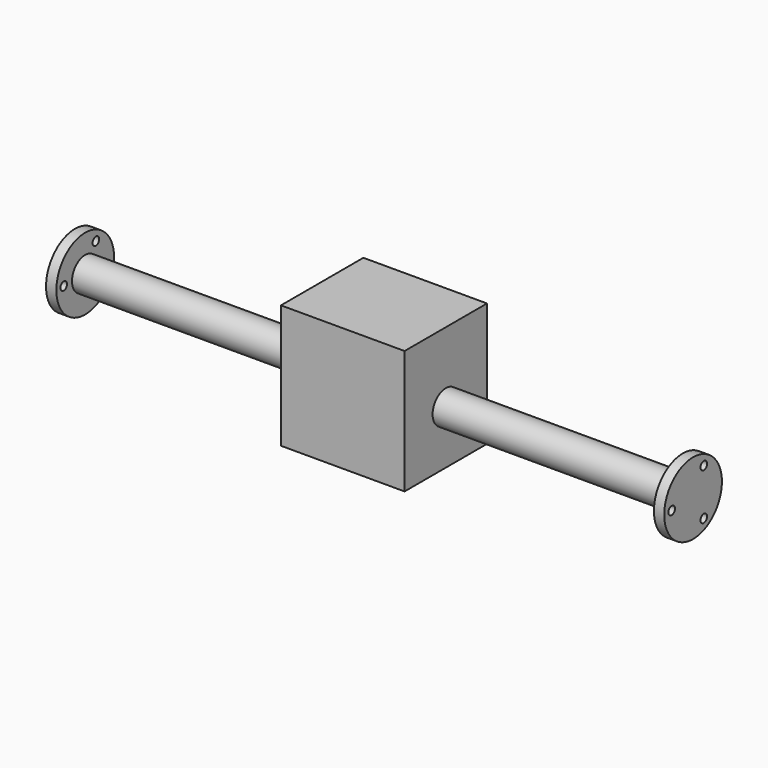
from build123d import *

# Parameters (mm, degrees)
F1_R            = 17.5
F2_DEPTH        = 5
F3_W            = 50
F3_H            = 60
F4_DEPTH        = 30
F5_R            = 8
F6_DEPTH        = 115
F7_R            = 2
F8_DEPTH        = 25
F8_COPIES_COUNT = 3


# Not quite as in the source:
# - a pattern or mirror of a feature is missing from the dataset's text; its kind, count and spacing are read off the source's solid


with BuildPart() as f2:
    # F1 (on offset) → F2 (new body)
    with BuildSketch(Plane.YZ.offset(150)):
        Circle(F1_R)
    extrude(amount=-F2_DEPTH)



with BuildPart() as f4:
    # F3 (on Right) → F4 (new body)
    with BuildSketch(Plane.YZ):
        with Locations((0, 4)):
            Rectangle(F3_W, F3_H)
    extrude(amount=F4_DEPTH)


with BuildPart() as f2_1:
    add(f2.part)

    add(f4.part)  # F6 merges F4
    # F5 (on face) → F6 (join, through all)
    with BuildSketch(Plane(origin=(145, 0, 0), x_dir=(0, -1, 0), z_dir=(-1, 0, 0))):
        Circle(F5_R)
    extrude(amount=F6_DEPTH)

    # F7 (on face) → F8 (cut)
    with BuildSketch(Plane.YZ.offset(150)):
        with Locations((-13, 0)):
            Circle(F7_R)
    f8 = extrude(amount=-F8_DEPTH, mode=Mode.SUBTRACT)

    # F8_copies: F8 ×3 about axis
    f8_copies_axis = Axis((0, 0, 0), (1, 0, 0))
    for i in range(1, F8_COPIES_COUNT):
        add(f8.rotate(f8_copies_axis, i * 360 / F8_COPIES_COUNT), mode=Mode.SUBTRACT)

    # F9: F2 across plane


with BuildPart() as f2_2:
    add(f2_1.part)
    add(f2_1.part.mirror(Plane.YZ))

    # F10: F2 across plane


with BuildPart() as f2_3:
    add(f2_2.part)
    add(f2_2.part.mirror(Plane.YZ))

    # F11: F2 across plane


with BuildPart() as f2_4:
    add(f2_3.part)
    add(f2_3.part.mirror(Plane.YZ))


solid = f2_4.part
